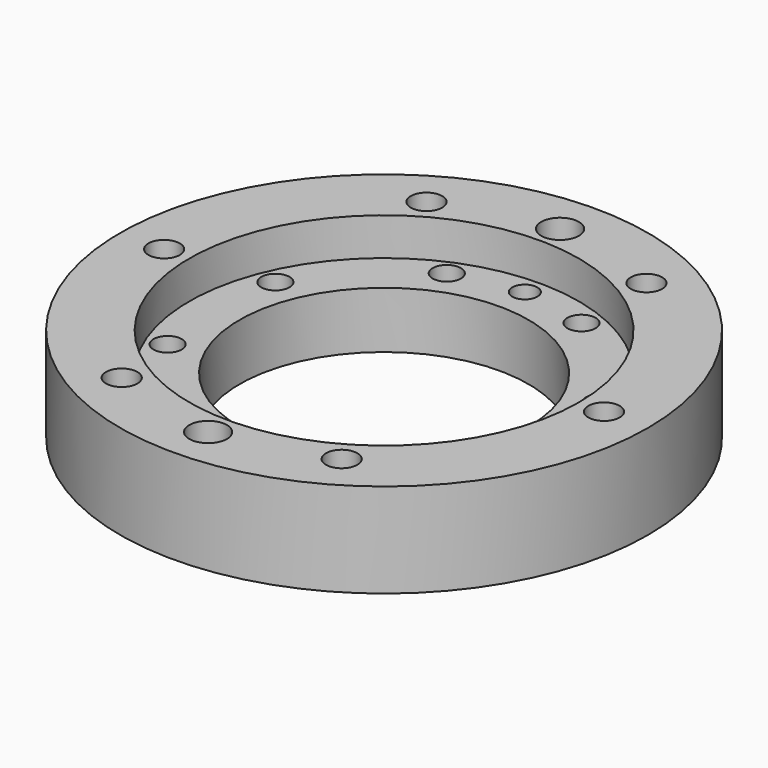
from build123d import *

# Parameters (mm, degrees)
F0_R             = 42
F0_R_2           = 23
F1_DEPTH         = 15
F2_R             = 31
F2_R_2           = 23
F3_DEPTH         = 6
F4_R             = 3
F5_DEPTH         = 15.001
F7_D             = 5
F7_COPIES_COUNT  = 6
F8_R             = 2
F9_DEPTH         = 15.001
F11_D            = 4.5
F11_CBORE_D      = 7.5
F11_CBORE_DEPTH  = 5.5
F11_COPIES_COUNT = 8


# Not quite as in the source:
# - a pattern or mirror of a feature is missing from the dataset's text; its kind, count and spacing are read off the source's solid


with BuildPart() as f1:
    # F0 (on Top) → F1 (new body)
    with BuildSketch(Plane.XY):
        Circle(F0_R)
        Circle(F0_R_2, mode=Mode.SUBTRACT)
    extrude(amount=-F1_DEPTH)

    # F2 (on face) → F3 (cut)
    with BuildSketch(Plane.XY):
        Circle(F2_R)
        Circle(F2_R_2, mode=Mode.SUBTRACT)
    extrude(amount=-F3_DEPTH, mode=Mode.SUBTRACT)

    # F4 (on face) → F5 (cut, through all)
    with BuildSketch(Plane.XY):
        with Locations((0, -35)):
            Circle(F4_R)
        with Locations((0, 35)):
            Circle(F4_R)
    extrude(amount=-F5_DEPTH, mode=Mode.SUBTRACT)

    # F7 (through all)
    with Locations(Plane.XY):
        with Locations((-17.5, 30.3108891325)):
            f7 = Hole(F7_D / 2)

    # F7_copies: F7 ×6 about axis
    f7_copies_axis = Axis((0, 0, 0), (0, 0, 1))
    for i in range(1, F7_COPIES_COUNT):
        add(f7.rotate(f7_copies_axis, i * 360 / F7_COPIES_COUNT), mode=Mode.SUBTRACT)

    # F8 (on face) → F9 (cut, through all)
    with BuildSketch(Plane(origin=(0, 0, -15), x_dir=(1, 0, 0), z_dir=(0, 0, -1))):
        with Locations((0, -28)):
            Circle(F8_R)
    extrude(amount=-F9_DEPTH, mode=Mode.SUBTRACT)

    # F11 (through all)
    with Locations(Plane(origin=(0, 0, -15), x_dir=(1, 0, 0), z_dir=(0, 0, -1))):
        with Locations((-10.7151361062, 25.8686269103)):
            f11 = CounterBoreHole(F11_D / 2, F11_CBORE_D / 2, F11_CBORE_DEPTH)

    # F11_copies: F11 ×8 about axis
    f11_copies_axis = Axis((0, 0, 0), (0, 0, 1))
    for i in range(1, F11_COPIES_COUNT):
        add(f11.rotate(f11_copies_axis, i * 360 / F11_COPIES_COUNT), mode=Mode.SUBTRACT)


solid = f1.part
